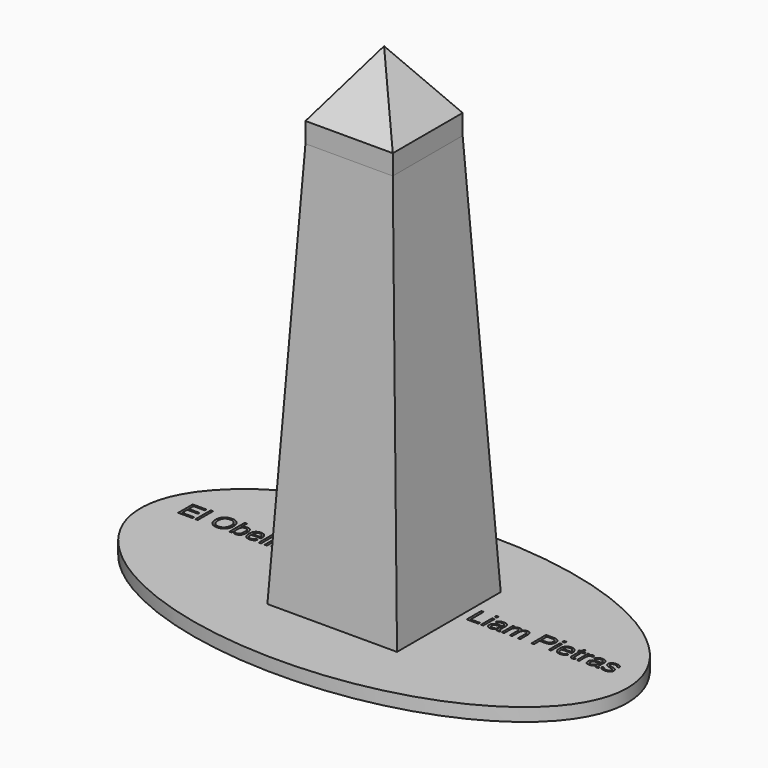
from build123d import *

# Parameters (mm, degrees)
F0_W          = 30
F0_H          = 30
F3_DEPTH      = 100
F3_TAPER      = 3
F2_W          = 20
F2_H          = 20
F4_DEPTH      = 15
F4_TAPER      = 35
F4_DEPTH_BACK = 25
F6_DEPTH      = 3
F7_TEXT_SIZE  = 6.0671558311
F8_DEPTH      = 1


# Not quite as in the source:
# - Text() gives the source's letters only with a copy of the font that has no kerning and outlines rounded to 1/6400 em; it was checked with that copy


with BuildPart() as f3:
    # F0 (on Top) → F3 (new body, through all)
    with BuildSketch(Plane.XY):
        Rectangle(F0_W, F0_H)
    extrude(amount=F3_DEPTH, taper=F3_TAPER)

    # F2 (on offset) → F4 (join, two sides)
    with BuildSketch(Plane.XY.offset(100)) as f4_sk:
        Rectangle(F2_W, F2_H)
    extrude(amount=F4_DEPTH, taper=F4_TAPER)
    extrude(f4_sk.sketch, amount=-F4_DEPTH_BACK)

    # F5 (on Top) → F6 (join)
    with BuildSketch(Plane.XY):
        with BuildLine():
            add(Edge.make_bspline(
                [(55.7436607778, 0), (55.7436607778, 53.0192894483), (-27.8718303889, 26.5096447242), (-111.4873215556, 0), (-27.8718303889, -26.5096447242), (55.7436607778, -53.0192894483), (55.7436607778, 0)],
                knots=[0, 0, 0, 2.0943951024, 2.0943951024, 4.1887902048, 4.1887902048, 6.2831853072, 6.2831853072, 6.2831853072], degree=2, weights=[1, 0.5, 1, 0.5, 1, 0.5, 1]))
        make_face()
    extrude(amount=F6_DEPTH)

    # F7 (on face) → F8 (cut)
    with BuildSketch(Plane.XY.offset(3)):
        with Locations((-49.8769918732, 2.7756542609)):
            Text('El Obelisco                     Liam Pietras', F7_TEXT_SIZE, font='Arimo', text_align=(TextAlign.LEFT, TextAlign.BOTTOM))
    extrude(amount=-F8_DEPTH, mode=Mode.SUBTRACT)


solid = f3.part
